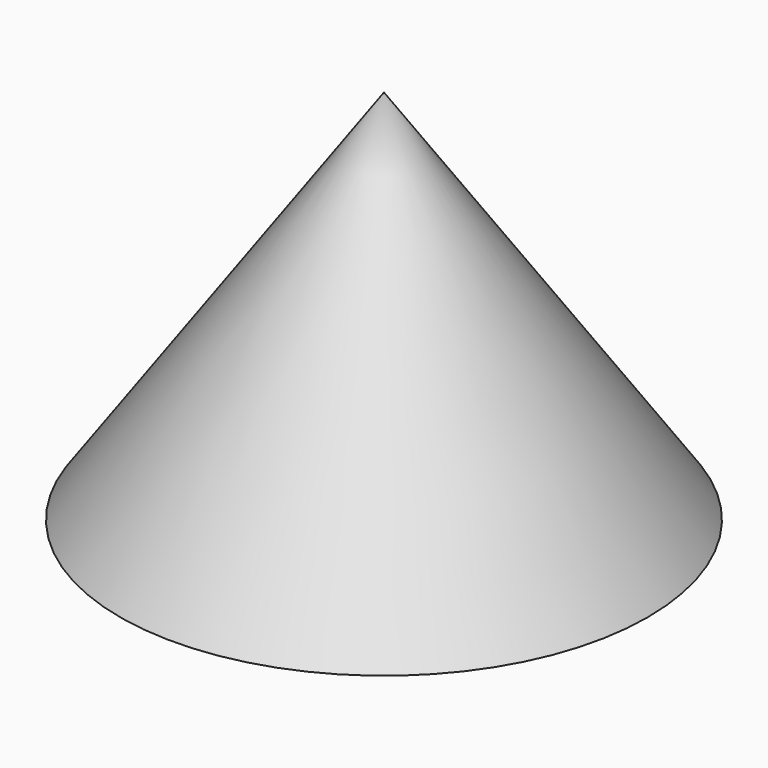
from build123d import *

# Parameters (mm, degrees)
F0_R = 17.8213876383


with BuildPart() as f3:
    # F0 (on Top) → F3 section 0
    with BuildSketch(Plane.XY, mode=Mode.PRIVATE) as f3_s0:
        Circle(F0_R)
    loft([f3_s0.sketch, Vertex(0, 0, 25.4)])


solid = f3.part
